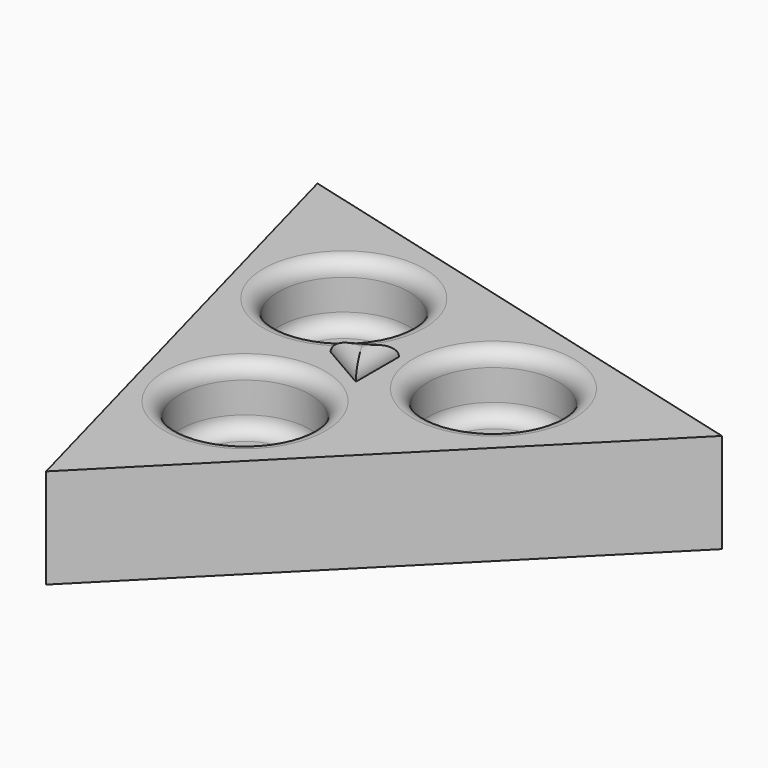
from build123d import *

# Parameters (mm, degrees)
F1_DEPTH = 33.02
F2_R     = 21.59
F3_DEPTH = 20.32
F4_R     = 5.08
F6_DEPTH = 5.08
F7_R     = 5.07999


# Not quite as in the source:
# - a fillet or chamfer is up to 0.001 mm smaller than in the source, because OpenCascade refuses the exact size


with BuildPart() as f1:
    # F0 (on Top) → F1 (new body)
    with BuildSketch(Plane.XY):
        Polygon((-26.044934144, -98.2049968455), (98.0704891188, 26.5469238142), (-72.0255549748, 71.6580730314), align=None)
    extrude(amount=F1_DEPTH)

    # F2 (on face) → F3 (cut)
    with BuildSketch(Plane.XY.offset(33.02)):
        with Locations((-26.4560222886, 25.6227981428)):
            Circle(F2_R)
        with Locations((-10.44000236, -35.3193325351)):
            Circle(F2_R)
        with Locations((35.3598029055, 10.3020987419)):
            Circle(F2_R)
    extrude(amount=-F3_DEPTH, mode=Mode.SUBTRACT)

    # F4
    f4_edges = [f1.edges().sort_by_distance(p)[0] for p in [
        (-48.046022, 25.622798, 33.02),
        (-32.030002, -35.319333, 33.02),
        (13.769803, 10.302099, 33.02),
        (-48.046022, 25.622798, 12.7),
        (-32.030002, -35.319333, 12.7),
        (13.769803, 10.302099, 12.7),
    ]]
    fillet(f4_edges, radius=F4_R)


with BuildPart() as f6:
    # F5 (on face) → F6 (new body)
    with BuildSketch(Plane.XY.offset(33.02)):
        Polygon((5.164898932, -8.9458673661), (5.164898932, 8.9458673661), (-10.329797864, 0), align=None)
    extrude(amount=F6_DEPTH)

    # F7 (radius 5.08 in the source; OpenCascade refuses exactly that, so slightly less here)
    f7_edges = [f6.edges().sort_by_distance(p)[0] for p in [
        (5.164899, 0, 38.1),
        (-2.582449, -4.472934, 38.1),
        (-2.582449, 4.472934, 38.1),
    ]]
    fillet(f7_edges, radius=F7_R)


solid = Compound([f1.part, f6.part])
